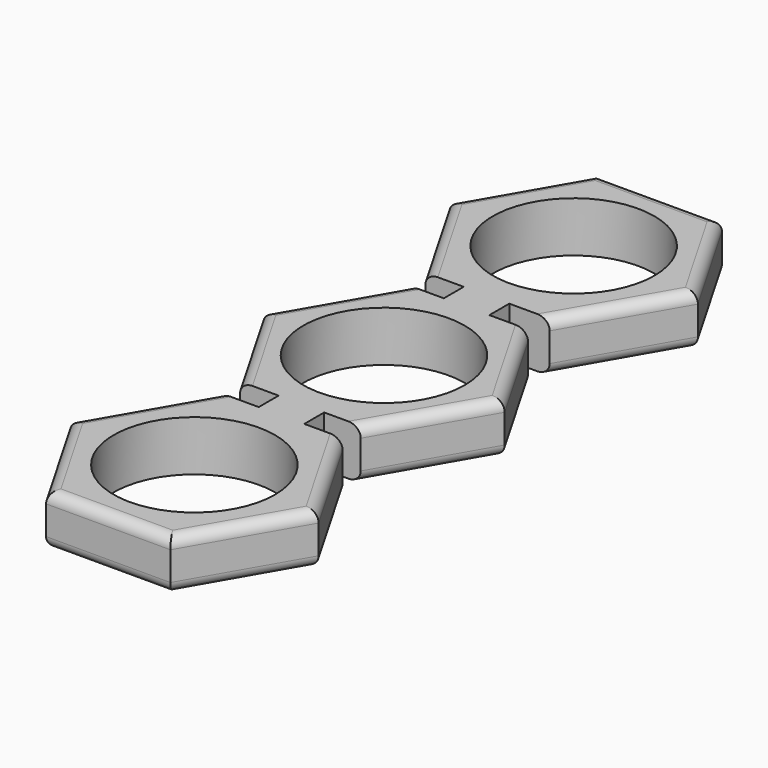
from build123d import *

# Parameters (mm, degrees)
F0_R     = 11.2
F0_W     = 6.3229973894
F0_H     = 3.449
F1_DEPTH = 7
F2_R     = 1.5


# Not quite as in the source:
# - ends of sketch curves that miss each other by under 0.0002 mm in the source are joined


with BuildPart() as f1:
    # F0 (on Top) → F1 (new body)
    with BuildSketch(Plane.XY):
        Polygon((-3.3052028157, 17.9631426474), (3.0177945737, 17.9631426474), (8.6286484148, 17.9631426474), (17.2572757273, 32.9083635521), (8.628630128, 47.8536161306), (-8.628630128, 47.8536161306), (-17.2572757273, 32.9083635521), (-8.6286484148, 17.9631426474), align=None)
        with Locations((0, 32.9083055258)):
            Circle(F0_R, mode=Mode.SUBTRACT)
        Polygon((3.3052028157, -14.5141426474), (8.3797441645, -14.5141426474), (16.759488329, 0), (8.3797441645, 14.5141426474), (3.0177945737, 14.5141426474), (-3.3052028157, 14.5141426474), (-8.3797441645, 14.5141426474), (-16.759488329, 0), (-8.3797441645, -14.5141426474), (-3.0177945737, -14.5141426474), align=None)
        Circle(F0_R, mode=Mode.SUBTRACT)
        with Locations((-0.143704121, 16.2386426474)):
            Rectangle(F0_W, F0_H)
        Polygon((8.6286484148, -17.9630480707), (3.3052028157, -17.9630480707), (-3.0177945737, -17.9630480707), (-8.6286484148, -17.9630480707), (-17.2572757273, -32.9082689754), (-8.628630128, -47.8535215539), (8.628630128, -47.8535215539), (17.2572757273, -32.9082689754), align=None)
        with Locations((0, -32.9082109491)):
            Circle(F0_R, mode=Mode.SUBTRACT)
        with Locations((0.143704121, -16.2386426474)):
            Rectangle(F0_W, F0_H)
    extrude(amount=F1_DEPTH)

    # F2
    f2_edges = [f1.edges().sort_by_distance(p)[0] for p in [
        (-12.942953, 40.38099, 7),
        (0, 47.853616, 7),
        (12.942953, 40.38099, 7),
        (12.942962, 25.435753, 7),
        (-12.942962, 25.435753, 7),
        (-12.569616, 7.257071, 7),
        (12.569616, -7.257071, 7),
        (-12.569616, -7.257071, 7),
        (-12.942962, -25.435659, 7),
        (12.942962, -25.435659, 7),
        (12.942953, -40.380895, 7),
        (0, -47.853522, 7),
        (-12.942953, -40.380895, 7),
        (12.569616, 7.257071, 7),
        (-12.942953, -40.380895, 0),
        (0, -47.853522, 0),
        (12.942953, -40.380895, 0),
        (12.942962, -25.435659, 0),
        (-12.942962, -25.435659, 0),
        (-12.569616, -7.257071, 0),
        (12.569616, -7.257071, 0),
        (12.569616, 7.257071, 0),
        (-12.569616, 7.257071, 0),
        (-12.942962, 25.435753, 0),
        (-12.942953, 40.38099, 0),
        (12.942953, 40.38099, 0),
        (0, 47.853616, 0),
        (12.942962, 25.435753, 0),
    ]]
    fillet(f2_edges, radius=F2_R)


solid = f1.part
